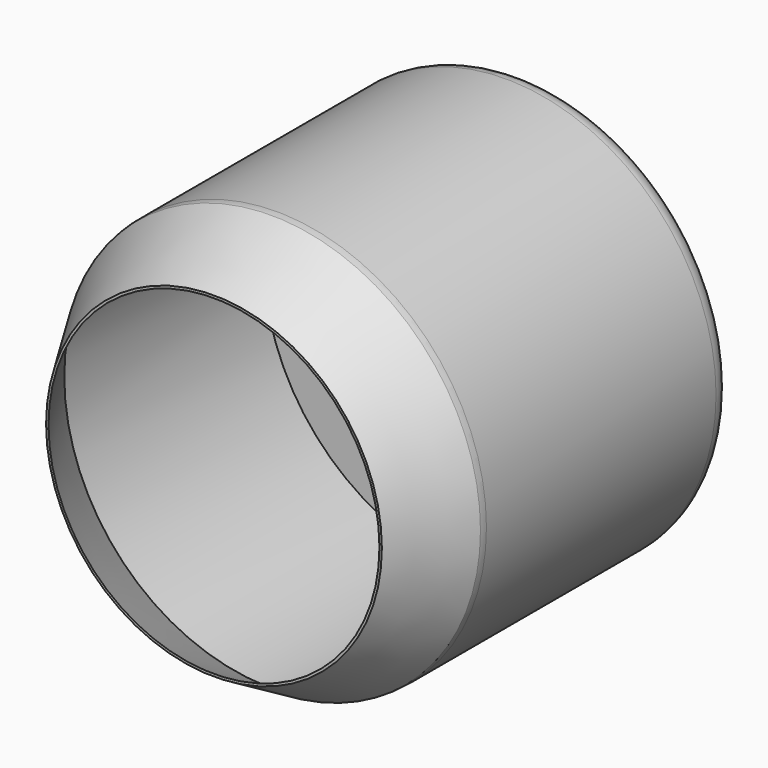
from build123d import *

# Parameters (mm, degrees)
F0_R     = 50
F1_DEPTH = 15
F2_R     = 50
F2_R_2   = 49.75
F3_DEPTH = 60
F6_R     = 5


# Not quite as in the source:
# - a fillet or chamfer that OpenCascade refuses, or shapes differently, is made with other operations: its cross-section is extruded or revolved along the edge and cut away or added


with BuildPart() as f1:
    # F0 (on Front) → F1 (new body)
    with BuildSketch(Plane.XZ):
        Circle(F0_R)
    extrude(amount=F1_DEPTH)

    # F2 (on face) → F3 (join)
    with BuildSketch(Plane.XZ.offset(15)):
        Circle(F2_R)
        Circle(F2_R_2, mode=Mode.SUBTRACT)
    extrude(amount=F3_DEPTH)

    # F4 (on Top) → F5 (revolve)
    with BuildSketch(Plane.XY):
        Polygon((-40, -92.0273140073), (-39.4221065602, -92.0273140073), (-49.289773818, -75), (-49.8676672578, -75), align=None)
    revolve(axis=Axis((0, -82.0273140073, 0), (0, -1, 0)))

    # F6
    f6_edges = [f1.edges().sort_by_distance(p)[0] for p in [
        (-50, 0, 0),
    ]]
    fillet(f6_edges, radius=F6_R)

    # F7: fillet of radius 10 on 1 edges, made by hand

    # F7_s1 → F7_t2 (revolve, cut)
    with BuildSketch(Plane.XY):
        with BuildLine():
            ThreePointArc((50, -73.378536806), (49.9668619078, -74.1919639453), (49.8676672578, -75))
            Line((49.8676672578, -75), (50, -75))
            Line((50, -75), (50, -73.378536806))
        make_face()
    revolve(axis=Axis((0, -75, 0), (0, -1, 0)), mode=Mode.SUBTRACT)


solid = f1.part
